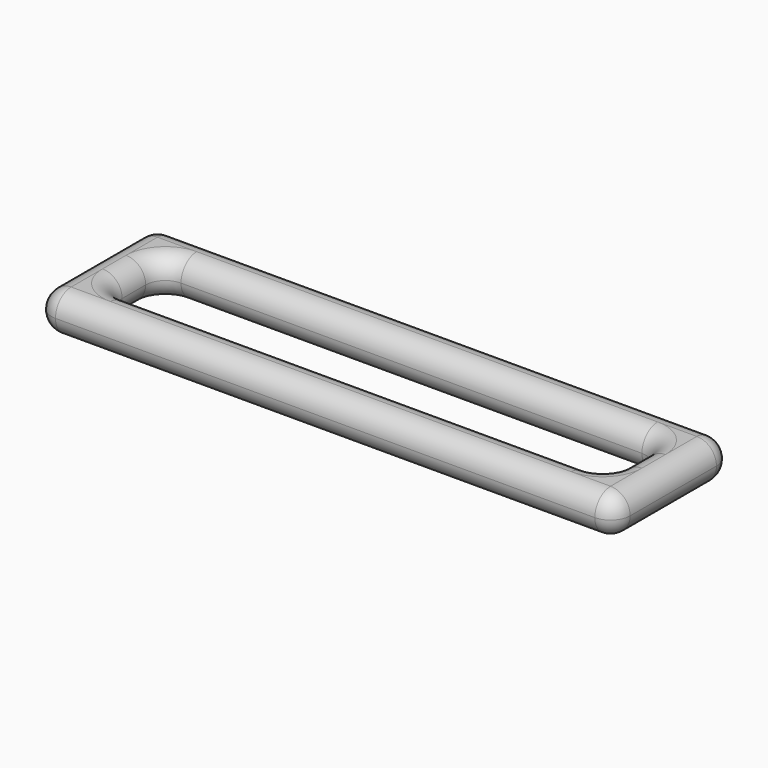
from build123d import *

# Parameters (mm, degrees)
F1_DEPTH = 2
F2_R     = 0.99999


# Not quite as in the source:
# - a fillet or chamfer is up to 0.001 mm smaller than in the source, because OpenCascade refuses the exact size


with BuildPart() as f1:
    # F0 (on Top) → F1 (new body)
    with BuildSketch(Plane.XY):
        with BuildLine():
            ThreePointArc((-13.75, 3.75), (-14.4571067812, 3.4571067812), (-14.75, 2.75))
            Line((-14.75, 2.75), (-14.75, -2.75))
            ThreePointArc((-14.75, -2.75), (-14.4571067812, -3.4571067812), (-13.75, -3.75))
            Line((-13.75, -3.75), (13.75, -3.75))
            ThreePointArc((13.75, -3.75), (14.4571067812, -3.4571067812), (14.75, -2.75))
            Line((14.75, -2.75), (14.75, 2.75))
            ThreePointArc((14.75, 2.75), (14.4571067812, 3.4571067812), (13.75, 3.75))
            Line((13.75, 3.75), (-13.75, 3.75))
        make_face()
        with BuildLine():
            Line((-11.75, 1.75), (11.75, 1.75))
            ThreePointArc((11.75, 1.75), (12.4571067812, 1.4571067812), (12.75, 0.75))
            Line((12.75, 0.75), (12.75, -0.75))
            ThreePointArc((12.75, -0.75), (12.4571067812, -1.4571067812), (11.75, -1.75))
            Line((11.75, -1.75), (-11.75, -1.75))
            ThreePointArc((-11.75, -1.75), (-12.4571067812, -1.4571067812), (-12.75, -0.75))
            Line((-12.75, -0.75), (-12.75, 0.75))
            ThreePointArc((-12.75, 0.75), (-12.4571067812, 1.4571067812), (-11.75, 1.75))
        make_face(mode=Mode.SUBTRACT)
    extrude(amount=F1_DEPTH)

    # F2 (radius 1 in the source; OpenCascade refuses exactly that, so slightly less here)
    f2_edges = [f1.edges().sort_by_distance(p)[0] for p in [
        (0, 1.75, 2),
        (0, 1.75, 0),
        (0, 3.75, 0),
        (0, -3.75, 2),
    ]]
    fillet(f2_edges, radius=F2_R)


solid = f1.part
